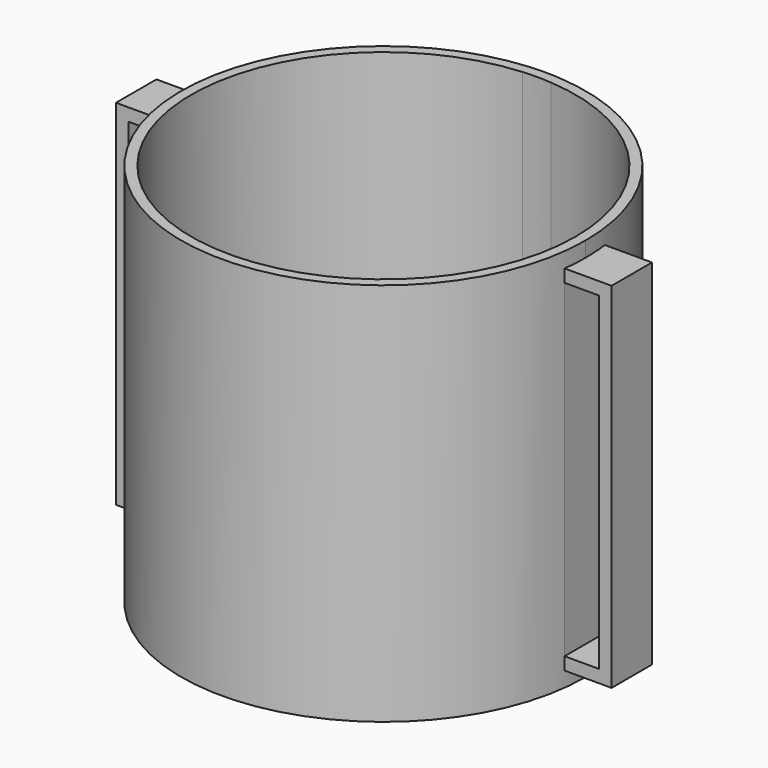
from build123d import *
from build123d import SkipClean  # not in build123d's __all__

# Parameters (mm, degrees)
F1_DEPTH = 38
F2_T     = -2
F3_W     = 10
F3_H     = 10
F4_DEPTH = 35
F5_W     = 6.789718
F5_H     = 65
F6_DEPTH = 25
F7_W     = 6.789718
F7_H     = 65
F8_DEPTH = 25


with BuildPart() as f1:
    # F0 (on Top) → F1 (new body, symmetric)
    with BuildSketch(Plane.XY):
        with BuildLine():
            ThreePointArc((-3, 39.887341), (-27.202941, -29.325757), (40, 0))
            ThreePointArc((40, 0), (29.325757, 27.202941), (3, 39.887341))
            ThreePointArc((3, 39.887341), (0, 40), (-3, 39.887341))
        make_face()
    extrude(amount=F1_DEPTH, both=True)

    # F2
    f2_openings = [f1.faces().sort_by_distance(p)[0] for p in [
        (0, 0, 38),
    ]]
    offset(amount=F2_T, openings=f2_openings)

    # F3 (on Top) → F4 (join, symmetric)
    with BuildSketch(Plane.XY):
        with Locations((-43.994746, 0.151211)):
            Rectangle(F3_W, F3_H)
        with Locations((43.994746, 0.151211)):
            Rectangle(F3_W, F3_H)
    with SkipClean():  # cleaning this boolean's faces spoils the solid; the shape is the same uncleaned
        extrude(amount=F4_DEPTH, both=True)

    # F5 (on face) → F6 (cut)
    with BuildSketch(Plane.XZ.offset(4.848789)):
        with Locations((-43.099887, 0)):
            Rectangle(F5_W, F5_H)
    with SkipClean():  # cleaning this boolean's faces spoils the solid; the shape is the same uncleaned
        extrude(amount=-F6_DEPTH, mode=Mode.SUBTRACT)

    # F7 (on face) → F8 (cut)
    with BuildSketch(Plane.XZ.offset(4.848789)):
        with Locations((43.099887, 0)):
            Rectangle(F7_W, F7_H)
    with SkipClean():  # cleaning this boolean's faces spoils the solid; the shape is the same uncleaned
        extrude(amount=-F8_DEPTH, mode=Mode.SUBTRACT)


solid = f1.part
